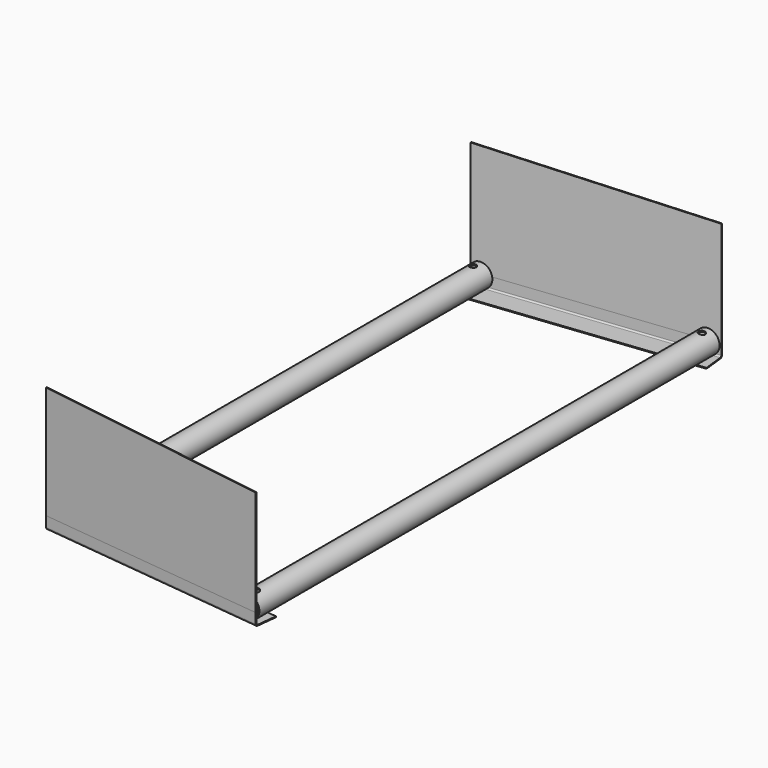
from build123d import *

# Parameters (mm, degrees)
F0_R      = 16
F0_R_2    = 14.4
F1_DEPTH  = 365
F2_R      = 16
F2_R_2    = 14.4
F3_DEPTH  = 397.5
F5_DEPTH  = 156
F7_DEPTH  = 320
F9_DEPTH  = 1.2
F11_R     = 4.5
F12_DEPTH = 18


with BuildPart() as f1:
    # F0 (on Front) → F1 (new body, symmetric)
    with BuildSketch(Plane.XZ):
        with Locations((-144, 0)):
            Circle(F0_R)
        with Locations((-144, 0)):
            Circle(F0_R_2, mode=Mode.SUBTRACT)
    extrude(amount=F1_DEPTH, both=True)


with BuildPart() as f3:
    # F2 (on Front) → F3 (new body, symmetric)
    with BuildSketch(Plane.XZ):
        with Locations((144, 0)):
            Circle(F2_R)
        with Locations((144, 0)):
            Circle(F2_R_2, mode=Mode.SUBTRACT)
    extrude(amount=F3_DEPTH, both=True)


with BuildPart() as f5:
    # F4 (on Top) → F5 (new body)
    with BuildSketch(Plane.XY):
        Polygon((159.1335545823, -401.614555292), (-158.8784003051, -366), (-159.0119548875, -367.1925448308), (159, -402.8071001228), align=None)
    extrude(amount=F5_DEPTH)

    # F6 (on face) → F7 (join)
    with BuildSketch(Plane(origin=(-116.4293426194, 13.0390672319, 0), x_dir=(-0.1112954853, -0.993787359, 0), z_dir=(-0.993787359, 0.1112954853, 0))):
        with BuildLine():
            Line((382.6086220662, 0), (381.4086220662, 0))
            Line((381.4086220662, 0), (381.4086220662, -14))
            ThreePointArc((381.4086220662, -14), (380.8228356286, -15.4142135624), (379.4086220662, -16))
            Line((379.4086220662, -16), (351.4086220662, -16))
            Line((351.4086220662, -16), (351.4086220662, -17.2))
            Line((351.4086220662, -17.2), (379.6086220662, -17.2))
            ThreePointArc((379.6086220662, -17.2), (381.7299424098, -16.3213203436), (382.6086220662, -14.2))
            Line((382.6086220662, -14.2), (382.6086220662, 0))
        make_face()
    extrude(amount=-F7_DEPTH)

    # F8 (on face) → F9 (cut, through all)
    with BuildSketch(Plane(origin=(-42.5826122681, -380.2316120627, 0), x_dir=(0.993787359, -0.1112954853, 0), z_dir=(-0.1112954853, -0.993787359, 0))):
        Polygon((202.8428017702, 156), (-117.1571982298, 156), (202.8428017702, 146), align=None)
    extrude(amount=-F9_DEPTH, mode=Mode.SUBTRACT)


with BuildPart() as f10_1:
    # F10: instance of F5
    add(f5.part.mirror(Plane.XZ))


with BuildPart() as f12_tool:
    # F11 (on Top) → F12 (new body, symmetric)
    with BuildSketch(Plane.XY):
        with Locations((-145.0119548875, -352.459148322)):
            Circle(F11_R)
        with Locations((145.3561455529, -384.977833891)):
            Circle(F11_R)
        with Locations((145.3561455529, 384.977833891)):
            Circle(F11_R)
        with Locations((-144.8784003051, 352.4741052662)):
            Circle(F11_R)
    extrude(amount=F12_DEPTH, both=True)


with BuildPart() as f1_1:
    add(f1.part)

    # F12: cut by f12_tool
    add(f12_tool.part, mode=Mode.SUBTRACT)


with BuildPart() as f3_1:
    add(f3.part)

    # F12: cut by f12_tool
    add(f12_tool.part, mode=Mode.SUBTRACT)


with BuildPart() as f5_1:
    add(f5.part)

    # F12: cut by f12_tool
    add(f12_tool.part, mode=Mode.SUBTRACT)


with BuildPart() as f10_1_1:
    add(f10_1.part)

    # F12: cut by f12_tool
    add(f12_tool.part, mode=Mode.SUBTRACT)


solid = Compound([f1_1.part, f3_1.part, f5_1.part, f10_1_1.part])
